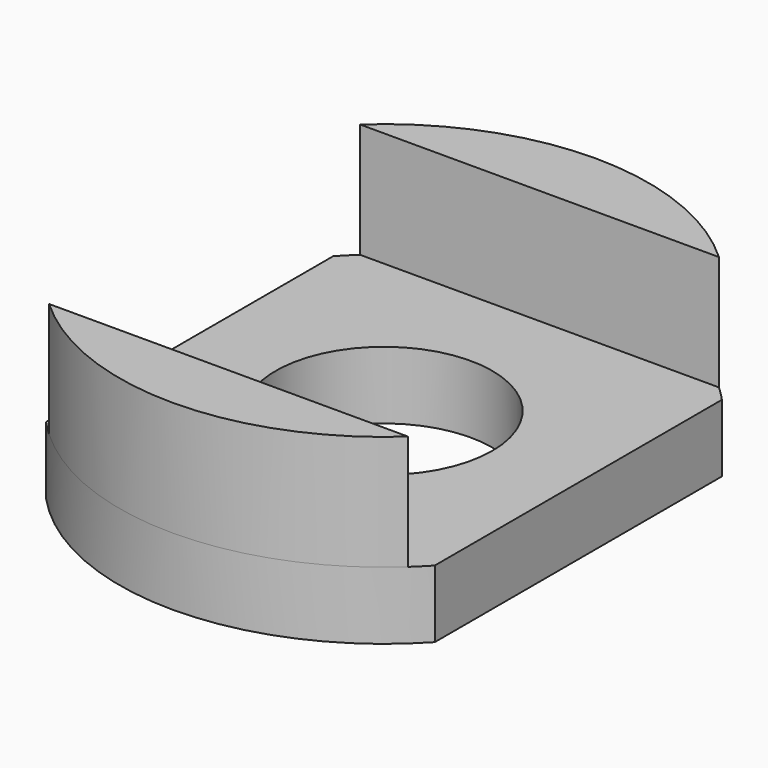
from build123d import *

# Parameters (mm, degrees)
F0_R     = 19.6
F0_R_2   = 8.025
F1_DEPTH = 5
F3_DEPTH = 8.5
F4_DEPTH = 5.001


with BuildPart() as f1:
    # F0 (on Top) → F1 (new body)
    with BuildSketch(Plane.XY):
        Circle(F0_R)
        Circle(F0_R_2, mode=Mode.SUBTRACT)
    extrude(amount=F1_DEPTH)

    # F2 (on face) → F3 (join)
    with BuildSketch(Plane.XY.offset(5)):
        with BuildLine():
            ThreePointArc((-13.2966161109, -14.4), (0, -19.6), (13.2966161109, -14.4))
            Line((13.2966161109, -14.4), (-13.2966161109, -14.4))
        make_face()
        with BuildLine():
            Line((-13.2966161109, 14.4), (13.2966161109, 14.4))
            ThreePointArc((13.2966161109, 14.4), (0, 19.6), (-13.2966161109, 14.4))
        make_face()
    extrude(amount=F3_DEPTH)

    # F2 (on face) → F4 (cut, through all)
    with BuildSketch(Plane.XY.offset(5)):
        with BuildLine():
            ThreePointArc((-14.4, 13.2966161109), (-19.6, 0), (-14.4, -13.2966161109))
            Line((-14.4, -13.2966161109), (-14.4, 13.2966161109))
        make_face()
        with BuildLine():
            Line((14.4, 13.2966161109), (14.4, -13.2966161109))
            ThreePointArc((14.4, -13.2966161109), (18.2537667346, -7.138627319), (19.6, 0))
            ThreePointArc((19.6, 0), (18.2537667346, 7.138627319), (14.4, 13.2966161109))
        make_face()
    extrude(amount=-F4_DEPTH, mode=Mode.SUBTRACT)


solid = f1.part
